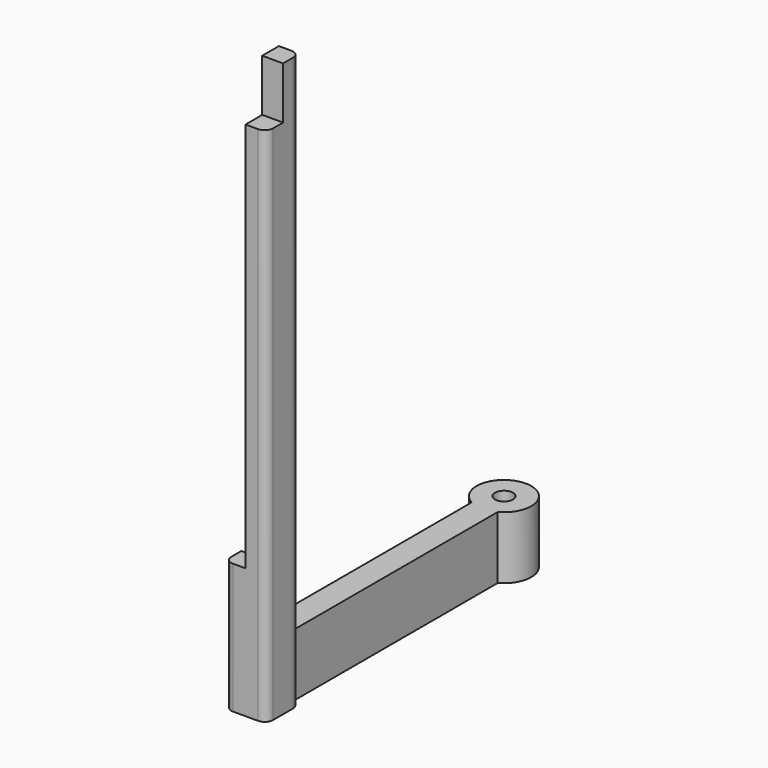
from build123d import *

# Parameters (mm, degrees)
F0_R     = 1.75
F1_DEPTH = 12
F2_DEPTH = 25
F4_DEPTH = 75
F6_DEPTH = 10
F8_DEPTH = 10


# Not quite as in the source:
# - a feature names something its author has since deleted; it is built from what else it names


with BuildPart() as f1:
    # F0 (on Top) → F1 (new body)
    with BuildSketch(Plane.XY):
        with BuildLine():
            ThreePointArc((2.5, -4.6165463282), (0, -5.25), (-2.5, -4.6165463282))
            Line((-2.5, -4.6165463282), (-2.5, -54))
            Line((-2.5, -54), (-2.4, -54))
            Line((-2.4, -54), (2.4, -54))
            Line((2.4, -54), (2.5, -54))
            Line((2.5, -54), (2.5, -4.6165463282))
        make_face()
        with BuildLine():
            Line((-2.5, -4), (-2.5, -4.6165463282))
            ThreePointArc((-2.5, -4.6165463282), (0, -5.25), (2.5, -4.6165463282))
            Line((2.5, -4.6165463282), (2.5, -4))
            Line((2.5, -4), (-2.5, -4))
        make_face()
        with BuildLine():
            ThreePointArc((2.5, -4.6165463282), (4.5104046382, -2.6867731575), (5.25, 0))
            ThreePointArc((5.25, 0), (-2.6867731575, 4.5104046382), (-2.5, -4.6165463282))
            Line((-2.5, -4.6165463282), (-2.5, -4))
            Line((-2.5, -4), (2.5, -4))
            Line((2.5, -4), (2.5, -4.6165463282))
        make_face()
        Circle(F0_R, mode=Mode.SUBTRACT)
    extrude(amount=F1_DEPTH)

    # F0 (on Top) → F2 (join)
    with BuildSketch(Plane.XY):
        with BuildLine():
            Line((2.4, -54), (-2.4, -54))
            ThreePointArc((-2.4, -54), (-3.5313708499, -54.4686291501), (-4, -55.6))
            Line((-4, -55.6), (-4, -60.4))
            ThreePointArc((-4, -60.4), (-3.5313708499, -61.5313708499), (-2.4, -62))
            Line((-2.4, -62), (2.4, -62))
            ThreePointArc((2.4, -62), (3.5313708499, -61.5313708499), (4, -60.4))
            Line((4, -60.4), (4, -55.6))
            ThreePointArc((4, -55.6), (3.5313708499, -54.4686291501), (2.4, -54))
        make_face()
    extrude(amount=F2_DEPTH)

    # F3 (on face) → F4 (join)
    with BuildSketch(Plane.XY.offset(25)):
        with BuildLine():
            Line((2.4, -54), (0, -54))
            Line((0, -54), (0, -62))
            Line((0, -62), (2.4, -62))
            ThreePointArc((2.4, -62), (3.5313708499, -61.5313708499), (4, -60.4))
            Line((4, -60.4), (4, -55.6))
            ThreePointArc((4, -55.6), (3.5313708499, -54.4686291501), (2.4, -54))
        make_face()
    extrude(amount=F4_DEPTH)

    # F5 (on face) → F6 (cut)
    with BuildSketch(Plane.XY.offset(25)):
        with BuildLine():
            Line((-4, -58), (0, -58))
            Line((0, -58), (0, -54))
            Line((0, -54), (-2.4, -54))
            ThreePointArc((-2.4, -54), (-3.5313708499, -54.4686291501), (-4, -55.6))
            Line((-4, -55.6), (-4, -58))
        make_face()
    extrude(amount=-F6_DEPTH, mode=Mode.SUBTRACT)

    # F7 (on face) → F8 (join)
    with BuildSketch(Plane.XY.offset(100)):
        with BuildLine():
            Line((0, -58), (4, -58))
            Line((4, -58), (4, -55.6))
            ThreePointArc((4, -55.6), (3.5313708499, -54.4686291501), (2.4, -54))
            Line((2.4, -54), (0, -54))
            Line((0, -54), (0, -58))
        make_face()
    extrude(amount=F8_DEPTH)


solid = f1.part
